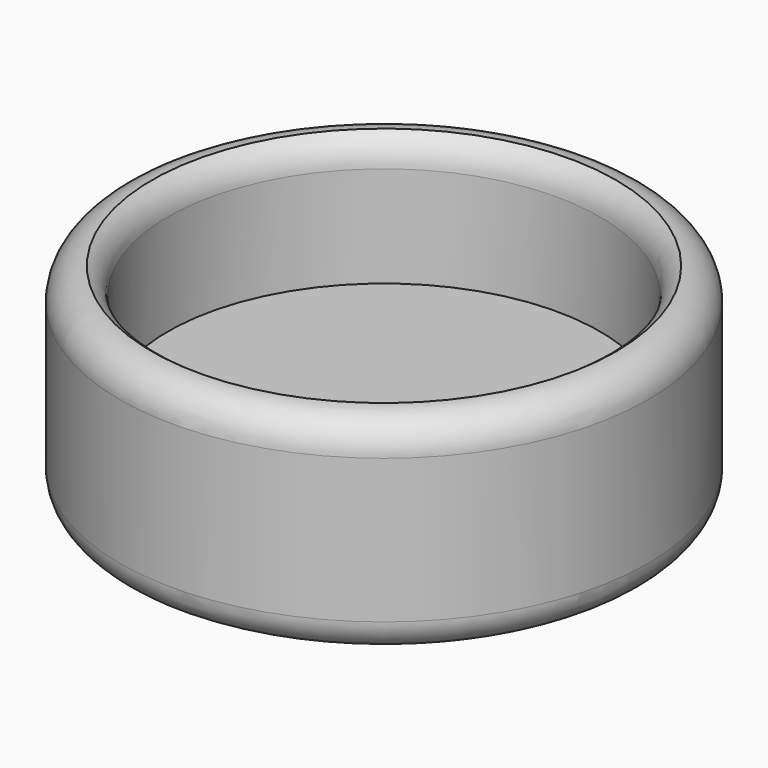
from build123d import *

# Parameters (mm, degrees)
F0_R     = 13.5
F1_DEPTH = 5
F0_R_2   = 16.5
F2_DEPTH = 13
F3_R     = 2


# Not quite as in the source:
# - a fillet or chamfer that OpenCascade refuses, or shapes differently, is made with other operations: its cross-section is extruded or revolved along the edge and cut away or added


with BuildPart() as f1:
    # F0 (on Top) → F1 (new body)
    with BuildSketch(Plane.XY):
        Circle(F0_R)
    extrude(amount=F1_DEPTH)

    # F0 (on Top) → F2 (join)
    with BuildSketch(Plane.XY):
        Circle(F0_R_2)
        Circle(F0_R, mode=Mode.SUBTRACT)
    extrude(amount=F2_DEPTH)

    # F3
    f3_edges = [f1.edges().sort_by_distance(p)[0] for p in [
        (-16.5, 0, 13),
        (-16.5, 0, 0),
    ]]
    fillet(f3_edges, radius=F3_R)

    # F4: fillet of radius 2 on 1 edges, made by hand

    # F4_s1 → F4_t2 (revolve, cut)
    with BuildSketch(Plane.XZ):
        with BuildLine():
            ThreePointArc((14.4997999035, 13.0003463544), (13.7675927526, 12.2678330874), (13.4996, 11.2673917434))
            Line((13.4996, 11.2673917434), (13.2994634315, 11.2673917434))
            ThreePointArc((13.2994634315, 11.2673917434), (13.2998634315, 12.1336958717), (13.2998634315, 13))
            Line((13.2998634315, 13), (13.5, 13.2001365685))
            ThreePointArc((13.5, 13.2001365685), (13.9998999517, 13.2001365685), (14.3996833253, 13.1736418155))
            Line((14.3996833253, 13.1736418155), (14.4997999035, 13.0003463544))
        make_face()
    revolve(axis=Axis((0, 0, 13), (0, 0, 1)), mode=Mode.SUBTRACT)


with BuildPart() as f5_1:
    # F5: copy of F1
    add(f1.part)


with BuildPart() as f7_1:
    # F7: copy of F1
    add(f1.part.moved(Location((0, 36, 0))))


with BuildPart() as f8_1:
    # F8: copy of F1
    add(f1.part.moved(Location((36.3, 0, 0))))


with BuildPart() as f9_1:
    # F9: copy of F8_1
    add(f8_1.part.moved(Location((-0.4, 35.2, 0))))


solid = f1.part
